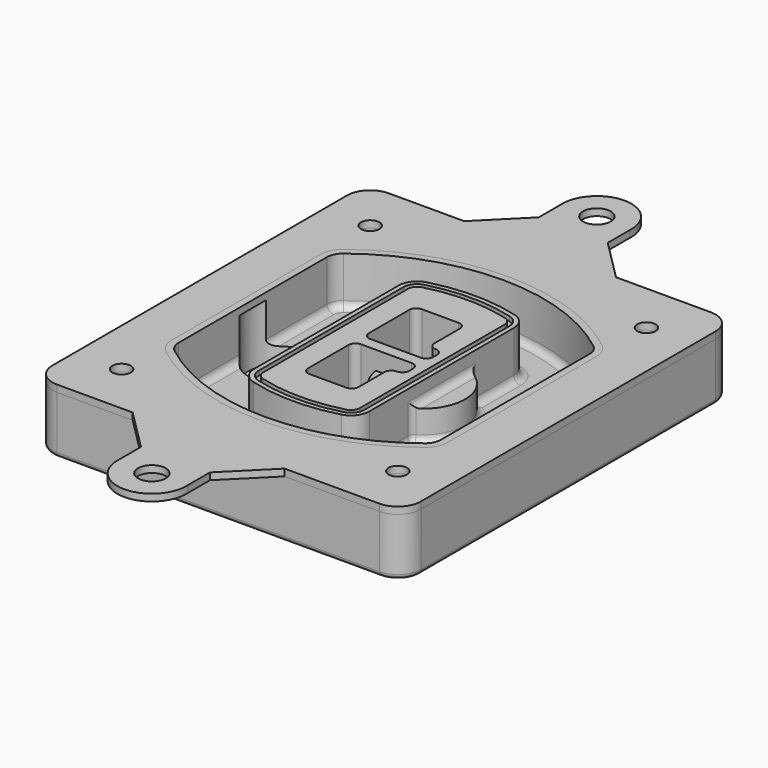
from build123d import *

# Parameters (mm, degrees)
F0_R      = 4
F1_DEPTH  = 25
F2_DEPTH  = 3
F3_DEPTH  = 18
F5_DEPTH  = 21
F6_DEPTH  = 2
F8_DEPTH  = 20
F9_DEPTH  = 16
F10_DEPTH = 25
F7_R      = 6
F7_R_2    = 4
F11_DEPTH = 6
F13_DEPTH = 9
F14_R     = 3
F15_R     = 2
F16_R     = 4
F16_R_2   = 6
F17_DEPTH = 3


# Not quite as in the source:
# - a feature names something its author has since deleted; it is built from what else it names


with BuildPart() as f1:
    # F0 (on Top) → F1 (new body)
    with BuildSketch(Plane.XY):
        with BuildLine():
            ThreePointArc((-80, -80), (-77.0710678119, -87.0710678119), (-70, -90))
            Line((-70, -90), (70, -90))
            ThreePointArc((70, -90), (77.0710678119, -87.0710678119), (80, -80))
            Line((80, -80), (80, 80))
            ThreePointArc((80, 80), (77.0710678119, 87.0710678119), (70, 90))
            Line((70, 90), (-70, 90))
            ThreePointArc((-70, 90), (-77.0710678119, 87.0710678119), (-80, 80))
            Line((-80, 80), (-80, -80))
        make_face()
        with Locations((-60, -67.5)):
            Circle(F0_R, mode=Mode.SUBTRACT)
        with Locations((60, -67.5)):
            Circle(F0_R, mode=Mode.SUBTRACT)
        with Locations((-60, 67.5)):
            Circle(F0_R, mode=Mode.SUBTRACT)
        with BuildLine():
            ThreePointArc((-64, 40.2934422872), (-62.5820384798, 46.4328484224), (-58.6153846154, 51.3286200352))
            ThreePointArc((-58.6153846154, 51.3286200352), (0, 71.5), (58.6153846154, 51.3286200352))
            ThreePointArc((58.6153846154, 51.3286200352), (62.5820384798, 46.4328484224), (64, 40.2934422872))
            Line((64, 40.2934422872), (64, -40.2934422872))
            ThreePointArc((64, -40.2934422872), (62.5820384798, -46.4328484224), (58.6153846154, -51.3286200352))
            ThreePointArc((58.6153846154, -51.3286200352), (0, -71.5), (-58.6153846154, -51.3286200352))
            ThreePointArc((-58.6153846154, -51.3286200352), (-62.5820384798, -46.4328484224), (-64, -40.2934422872))
            Line((-64, -40.2934422872), (-64, 40.2934422872))
        make_face(mode=Mode.SUBTRACT)
        with Locations((60, 67.5)):
            Circle(F0_R, mode=Mode.SUBTRACT)
        with BuildLine():
            ThreePointArc((58.6153846154, 51.3286200352), (0, 71.5), (-58.6153846154, 51.3286200352))
            ThreePointArc((-58.6153846154, 51.3286200352), (-62.5820384798, 46.4328484224), (-64, 40.2934422872))
            Line((-64, 40.2934422872), (-64, -40.2934422872))
            ThreePointArc((-64, -40.2934422872), (-62.5820384798, -46.4328484224), (-58.6153846154, -51.3286200352))
            ThreePointArc((-58.6153846154, -51.3286200352), (0, -71.5), (58.6153846154, -51.3286200352))
            ThreePointArc((58.6153846154, -51.3286200352), (62.5820384798, -46.4328484224), (64, -40.2934422872))
            Line((64, -40.2934422872), (64, 40.2934422872))
            ThreePointArc((64, 40.2934422872), (62.5820384798, 46.4328484224), (58.6153846154, 51.3286200352))
        make_face()
        with BuildLine():
            Line((-60, -40.2934422872), (-60, 40.2934422872))
            ThreePointArc((-60, 40.2934422872), (-58.9871703427, 44.6787323838), (-56.1538461538, 48.1757121072))
            ThreePointArc((-56.1538461538, 48.1757121072), (0, 67.5), (56.1538461538, 48.1757121072))
            ThreePointArc((56.1538461538, 48.1757121072), (58.9871703427, 44.6787323838), (60, 40.2934422872))
            Line((60, 40.2934422872), (60, -40.2934422872))
            ThreePointArc((60, -40.2934422872), (58.9871703427, -44.6787323838), (56.1538461538, -48.1757121072))
            ThreePointArc((56.1538461538, -48.1757121072), (0, -67.5), (-56.1538461538, -48.1757121072))
            ThreePointArc((-56.1538461538, -48.1757121072), (-58.9871703427, -44.6787323838), (-60, -40.2934422872))
        make_face(mode=Mode.SUBTRACT)
        with BuildLine():
            ThreePointArc((-56.1538461538, 48.1757121072), (-58.9871703427, 44.6787323838), (-60, 40.2934422872))
            Line((-60, 40.2934422872), (-60, -40.2934422872))
            ThreePointArc((-60, -40.2934422872), (-58.9871703427, -44.6787323838), (-56.1538461538, -48.1757121072))
            ThreePointArc((-56.1538461538, -48.1757121072), (0, -67.5), (56.1538461538, -48.1757121072))
            ThreePointArc((56.1538461538, -48.1757121072), (58.9871703427, -44.6787323838), (60, -40.2934422872))
            Line((60, -40.2934422872), (60, 40.2934422872))
            ThreePointArc((60, 40.2934422872), (58.9871703427, 44.6787323838), (56.1538461538, 48.1757121072))
            ThreePointArc((56.1538461538, 48.1757121072), (0, 67.5), (-56.1538461538, 48.1757121072))
        make_face()
        with BuildLine():
            ThreePointArc((54.3076923077, 45.8110311612), (56.2910192399, 43.3631453548), (57, 40.2934422872))
            Line((57, 40.2934422872), (57, -40.2934422872))
            ThreePointArc((57, -40.2934422872), (56.2910192399, -43.3631453548), (54.3076923077, -45.8110311612))
            ThreePointArc((54.3076923077, -45.8110311612), (0, -64.5), (-54.3076923077, -45.8110311612))
            ThreePointArc((-54.3076923077, -45.8110311612), (-56.2910192399, -43.3631453548), (-57, -40.2934422872))
            Line((-57, -40.2934422872), (-57, 40.2934422872))
            ThreePointArc((-57, 40.2934422872), (-56.2910192399, 43.3631453548), (-54.3076923077, 45.8110311612))
            ThreePointArc((-54.3076923077, 45.8110311612), (0, 64.5), (54.3076923077, 45.8110311612))
        make_face(mode=Mode.SUBTRACT)
        with BuildLine():
            Line((57, -40.2934422872), (57, 40.2934422872))
            ThreePointArc((57, 40.2934422872), (56.2910192399, 43.3631453548), (54.3076923077, 45.8110311612))
            ThreePointArc((54.3076923077, 45.8110311612), (0, 64.5), (-54.3076923077, 45.8110311612))
            ThreePointArc((-54.3076923077, 45.8110311612), (-56.2910192399, 43.3631453548), (-57, 40.2934422872))
            Line((-57, 40.2934422872), (-57, -40.2934422872))
            ThreePointArc((-57, -40.2934422872), (-56.2910192399, -43.3631453548), (-54.3076923077, -45.8110311612))
            ThreePointArc((-54.3076923077, -45.8110311612), (0, -64.5), (54.3076923077, -45.8110311612))
            ThreePointArc((54.3076923077, -45.8110311612), (56.2910192399, -43.3631453548), (57, -40.2934422872))
        make_face()
    extrude(amount=-F1_DEPTH)

    # F0 (on Top) → F2 (join)
    with BuildSketch(Plane.XY):
        with BuildLine():
            ThreePointArc((-56.1538461538, 48.1757121072), (-58.9871703427, 44.6787323838), (-60, 40.2934422872))
            Line((-60, 40.2934422872), (-60, -40.2934422872))
            ThreePointArc((-60, -40.2934422872), (-58.9871703427, -44.6787323838), (-56.1538461538, -48.1757121072))
            ThreePointArc((-56.1538461538, -48.1757121072), (0, -67.5), (56.1538461538, -48.1757121072))
            ThreePointArc((56.1538461538, -48.1757121072), (58.9871703427, -44.6787323838), (60, -40.2934422872))
            Line((60, -40.2934422872), (60, 40.2934422872))
            ThreePointArc((60, 40.2934422872), (58.9871703427, 44.6787323838), (56.1538461538, 48.1757121072))
            ThreePointArc((56.1538461538, 48.1757121072), (0, 67.5), (-56.1538461538, 48.1757121072))
        make_face()
        with BuildLine():
            ThreePointArc((54.3076923077, 45.8110311612), (56.2910192399, 43.3631453548), (57, 40.2934422872))
            Line((57, 40.2934422872), (57, -40.2934422872))
            ThreePointArc((57, -40.2934422872), (56.2910192399, -43.3631453548), (54.3076923077, -45.8110311612))
            ThreePointArc((54.3076923077, -45.8110311612), (0, -64.5), (-54.3076923077, -45.8110311612))
            ThreePointArc((-54.3076923077, -45.8110311612), (-56.2910192399, -43.3631453548), (-57, -40.2934422872))
            Line((-57, -40.2934422872), (-57, 40.2934422872))
            ThreePointArc((-57, 40.2934422872), (-56.2910192399, 43.3631453548), (-54.3076923077, 45.8110311612))
            ThreePointArc((-54.3076923077, 45.8110311612), (0, 64.5), (54.3076923077, 45.8110311612))
        make_face(mode=Mode.SUBTRACT)
    extrude(amount=F2_DEPTH)

    # F0 (on Top) → F3 (cut)
    with BuildSketch(Plane.XY):
        with BuildLine():
            Line((57, -40.2934422872), (57, 40.2934422872))
            ThreePointArc((57, 40.2934422872), (56.2910192399, 43.3631453548), (54.3076923077, 45.8110311612))
            ThreePointArc((54.3076923077, 45.8110311612), (0, 64.5), (-54.3076923077, 45.8110311612))
            ThreePointArc((-54.3076923077, 45.8110311612), (-56.2910192399, 43.3631453548), (-57, 40.2934422872))
            Line((-57, 40.2934422872), (-57, -40.2934422872))
            ThreePointArc((-57, -40.2934422872), (-56.2910192399, -43.3631453548), (-54.3076923077, -45.8110311612))
            ThreePointArc((-54.3076923077, -45.8110311612), (0, -64.5), (54.3076923077, -45.8110311612))
            ThreePointArc((54.3076923077, -45.8110311612), (56.2910192399, -43.3631453548), (57, -40.2934422872))
        make_face()
    extrude(amount=-F3_DEPTH, mode=Mode.SUBTRACT)

    # F4 (on face) → F5 (join, through all)
    with BuildSketch(Plane.XY.offset(3)):
        with BuildLine():
            ThreePointArc((-25, -39.2465276821), (-23.3511545998, -44.1109737193), (-19.0842911877, -46.9702398883))
            ThreePointArc((-19.0842911877, -46.9702398883), (0, -49.5), (19.0842911877, -46.9702398883))
            ThreePointArc((19.0842911877, -46.9702398883), (23.3511545998, -44.1109737193), (25, -39.2465276821))
            Line((25, -39.2465276821), (25, 39.2465276821))
            ThreePointArc((25, 39.2465276821), (23.3511545998, 44.1109737193), (19.0842911877, 46.9702398883))
            ThreePointArc((19.0842911877, 46.9702398883), (0, 49.5), (-19.0842911877, 46.9702398883))
            ThreePointArc((-19.0842911877, 46.9702398883), (-23.3511545998, 44.1109737193), (-25, 39.2465276821))
            Line((-25, 39.2465276821), (-25, -39.2465276821))
        make_face()
        with BuildLine():
            ThreePointArc((18.5632183908, 45.0393118368), (21.7633659499, 42.89486221), (23, 39.2465276821))
            Line((23, 39.2465276821), (23, -39.2465276821))
            ThreePointArc((23, -39.2465276821), (21.7633659499, -42.89486221), (18.5632183908, -45.0393118368))
            ThreePointArc((18.5632183908, -45.0393118368), (0, -47.5), (-18.5632183908, -45.0393118368))
            ThreePointArc((-18.5632183908, -45.0393118368), (-21.7633659499, -42.89486221), (-23, -39.2465276821))
            Line((-23, -39.2465276821), (-23, 39.2465276821))
            ThreePointArc((-23, 39.2465276821), (-21.7633659499, 42.89486221), (-18.5632183908, 45.0393118368))
            ThreePointArc((-18.5632183908, 45.0393118368), (0, 47.5), (18.5632183908, 45.0393118368))
        make_face(mode=Mode.SUBTRACT)
        with BuildLine():
            Line((23, -39.2465276821), (23, 39.2465276821))
            ThreePointArc((23, 39.2465276821), (21.7633659499, 42.89486221), (18.5632183908, 45.0393118368))
            ThreePointArc((18.5632183908, 45.0393118368), (0, 47.5), (-18.5632183908, 45.0393118368))
            ThreePointArc((-18.5632183908, 45.0393118368), (-21.7633659499, 42.89486221), (-23, 39.2465276821))
            Line((-23, 39.2465276821), (-23, -39.2465276821))
            ThreePointArc((-23, -39.2465276821), (-21.7633659499, -42.89486221), (-18.5632183908, -45.0393118368))
            ThreePointArc((-18.5632183908, -45.0393118368), (0, -47.5), (18.5632183908, -45.0393118368))
            ThreePointArc((18.5632183908, -45.0393118368), (21.7633659499, -42.89486221), (23, -39.2465276821))
        make_face()
        with BuildLine():
            ThreePointArc((18.0421455939, 43.1083837852), (20.1755772999, 41.6787507007), (21, 39.2465276821))
            Line((21, 39.2465276821), (21, -39.2465276821))
            ThreePointArc((21, -39.2465276821), (20.1755772999, -41.6787507007), (18.0421455939, -43.1083837852))
            ThreePointArc((18.0421455939, -43.1083837852), (0, -45.5), (-18.0421455939, -43.1083837852))
            ThreePointArc((-18.0421455939, -43.1083837852), (-20.1755772999, -41.6787507007), (-21, -39.2465276821))
            Line((-21, -39.2465276821), (-21, 39.2465276821))
            ThreePointArc((-21, 39.2465276821), (-20.1755772999, 41.6787507007), (-18.0421455939, 43.1083837852))
            ThreePointArc((-18.0421455939, 43.1083837852), (0, 45.5), (18.0421455939, 43.1083837852))
        make_face(mode=Mode.SUBTRACT)
        with BuildLine():
            Line((21, -39.2465276821), (21, 39.2465276821))
            ThreePointArc((21, 39.2465276821), (20.1755772999, 41.6787507007), (18.0421455939, 43.1083837852))
            ThreePointArc((18.0421455939, 43.1083837852), (0, 45.5), (-18.0421455939, 43.1083837852))
            ThreePointArc((-18.0421455939, 43.1083837852), (-20.1755772999, 41.6787507007), (-21, 39.2465276821))
            Line((-21, 39.2465276821), (-21, -39.2465276821))
            ThreePointArc((-21, -39.2465276821), (-20.1755772999, -41.6787507007), (-18.0421455939, -43.1083837852))
            ThreePointArc((-18.0421455939, -43.1083837852), (0, -45.5), (18.0421455939, -43.1083837852))
            ThreePointArc((18.0421455939, -43.1083837852), (20.1755772999, -41.6787507007), (21, -39.2465276821))
        make_face()
        with BuildLine():
            Line((-8, -2.5), (14, -2.5))
            ThreePointArc((14, -2.5), (16.1213203436, -3.3786796564), (17, -5.5))
            Line((17, -5.5), (17, -7.5))
            ThreePointArc((17, -7.5), (16.1213203436, -9.6213203436), (14, -10.5))
            ThreePointArc((14, -10.5), (11.8786796564, -11.3786796564), (11, -13.5))
            Line((11, -13.5), (11, -27.5))
            ThreePointArc((11, -27.5), (10.1213203436, -29.6213203436), (8, -30.5))
            Line((8, -30.5), (-8, -30.5))
            ThreePointArc((-8, -30.5), (-10.1213203436, -29.6213203436), (-11, -27.5))
            Line((-11, -27.5), (-11, -5.5))
            ThreePointArc((-11, -5.5), (-10.1213203436, -3.3786796564), (-8, -2.5))
        make_face(mode=Mode.SUBTRACT)
        with BuildLine():
            ThreePointArc((-8, 2.5), (-10.1213203436, 3.3786796564), (-11, 5.5))
            Line((-11, 5.5), (-11, 27.5))
            ThreePointArc((-11, 27.5), (-10.1213203436, 29.6213203436), (-8, 30.5))
            Line((-8, 30.5), (8, 30.5))
            ThreePointArc((8, 30.5), (10.1213203436, 29.6213203436), (11, 27.5))
            Line((11, 27.5), (11, 13.5))
            ThreePointArc((11, 13.5), (11.8786796564, 11.3786796564), (14, 10.5))
            ThreePointArc((14, 10.5), (16.1213203436, 9.6213203436), (17, 7.5))
            Line((17, 7.5), (17, 5.5))
            ThreePointArc((17, 5.5), (16.1213203436, 3.3786796564), (14, 2.5))
            Line((14, 2.5), (-8, 2.5))
        make_face(mode=Mode.SUBTRACT)
    extrude(amount=-F5_DEPTH)

    # F4 (on face) → F6 (cut)
    with BuildSketch(Plane.XY.offset(3)):
        with BuildLine():
            Line((23, -39.2465276821), (23, 39.2465276821))
            ThreePointArc((23, 39.2465276821), (21.7633659499, 42.89486221), (18.5632183908, 45.0393118368))
            ThreePointArc((18.5632183908, 45.0393118368), (0, 47.5), (-18.5632183908, 45.0393118368))
            ThreePointArc((-18.5632183908, 45.0393118368), (-21.7633659499, 42.89486221), (-23, 39.2465276821))
            Line((-23, 39.2465276821), (-23, -39.2465276821))
            ThreePointArc((-23, -39.2465276821), (-21.7633659499, -42.89486221), (-18.5632183908, -45.0393118368))
            ThreePointArc((-18.5632183908, -45.0393118368), (0, -47.5), (18.5632183908, -45.0393118368))
            ThreePointArc((18.5632183908, -45.0393118368), (21.7633659499, -42.89486221), (23, -39.2465276821))
        make_face()
        with BuildLine():
            ThreePointArc((18.0421455939, 43.1083837852), (20.1755772999, 41.6787507007), (21, 39.2465276821))
            Line((21, 39.2465276821), (21, -39.2465276821))
            ThreePointArc((21, -39.2465276821), (20.1755772999, -41.6787507007), (18.0421455939, -43.1083837852))
            ThreePointArc((18.0421455939, -43.1083837852), (0, -45.5), (-18.0421455939, -43.1083837852))
            ThreePointArc((-18.0421455939, -43.1083837852), (-20.1755772999, -41.6787507007), (-21, -39.2465276821))
            Line((-21, -39.2465276821), (-21, 39.2465276821))
            ThreePointArc((-21, 39.2465276821), (-20.1755772999, 41.6787507007), (-18.0421455939, 43.1083837852))
            ThreePointArc((-18.0421455939, 43.1083837852), (0, 45.5), (18.0421455939, 43.1083837852))
        make_face(mode=Mode.SUBTRACT)
    extrude(amount=-F6_DEPTH, mode=Mode.SUBTRACT)

    # F7 (on face) → F8 (join)
    with BuildSketch(Plane(origin=(0, 0, -25), x_dir=(1, 0, 0), z_dir=(0, 0, -1))):
        with BuildLine():
            ThreePointArc((3.28842436, 0), (16.7567035675, 13.4682792075), (30.224982775, 0))
            Line((30.224982775, 0), (35.224982775, 0))
            ThreePointArc((35.224982775, 0), (16.7567035675, 18.4682792075), (-1.71157564, 0))
            Line((-1.71157564, 0), (3.28842436, 0))
        make_face()
        with BuildLine():
            Line((3.28842436, 0), (30.224982775, 0))
            ThreePointArc((30.224982775, 0), (16.7567035675, 13.4682792075), (3.28842436, 0))
        make_face()
        with BuildLine():
            ThreePointArc((3.28842436, 0), (16.7567035675, -13.4682792075), (30.224982775, 0))
            Line((30.224982775, 0), (3.28842436, 0))
        make_face()
        with BuildLine():
            Line((35.224982775, 0), (30.224982775, 0))
            ThreePointArc((30.224982775, 0), (16.7567035675, -13.4682792075), (3.28842436, 0))
            Line((3.28842436, 0), (-1.71157564, 0))
            ThreePointArc((-1.71157564, 0), (16.7567035675, -18.4682792075), (35.224982775, 0))
        make_face()
    extrude(amount=-F8_DEPTH)

    # F7 (on face) → F9 (cut)
    with BuildSketch(Plane(origin=(0, 0, -25), x_dir=(1, 0, 0), z_dir=(0, 0, -1))):
        with BuildLine():
            Line((3.28842436, 0), (30.224982775, 0))
            ThreePointArc((30.224982775, 0), (16.7567035675, 13.4682792075), (3.28842436, 0))
        make_face()
        with BuildLine():
            ThreePointArc((3.28842436, 0), (16.7567035675, -13.4682792075), (30.224982775, 0))
            Line((30.224982775, 0), (3.28842436, 0))
        make_face()
    extrude(amount=-F9_DEPTH, mode=Mode.SUBTRACT)

    # F7 (on face) → F10 (cut)
    with BuildSketch(Plane(origin=(0, 0, -25), x_dir=(1, 0, 0), z_dir=(0, 0, -1))):
        with BuildLine():
            Line((-59.0318229325, 0), (-32.0952645175, 0))
            ThreePointArc((-32.0952645175, 0), (-45.563543725, 13.4682792075), (-59.0318229325, 0))
        make_face()
        with BuildLine():
            ThreePointArc((-59.0318229325, 0), (-45.563543725, -13.4682792075), (-32.0952645175, 0))
            Line((-32.0952645175, 0), (-59.0318229325, 0))
        make_face()
    extrude(amount=-F10_DEPTH, mode=Mode.SUBTRACT)

    # F7 (on face) → F11 (cut)
    with BuildSketch(Plane(origin=(0, 0, -25), x_dir=(1, 0, 0), z_dir=(0, 0, -1))):
        with Locations((60, -67.5)):
            Circle(F7_R)
        with Locations((60, -67.5)):
            Circle(F7_R_2, mode=Mode.SUBTRACT)
        with Locations((-60, -67.5)):
            Circle(F7_R)
        with Locations((-60, -67.5)):
            Circle(F7_R_2, mode=Mode.SUBTRACT)
        with Locations((-60, 67.5)):
            Circle(F7_R)
        with Locations((-60, 67.5)):
            Circle(F7_R_2, mode=Mode.SUBTRACT)
        with Locations((60, 67.5)):
            Circle(F7_R)
        with Locations((60, 67.5)):
            Circle(F7_R_2, mode=Mode.SUBTRACT)
    extrude(amount=-F11_DEPTH, mode=Mode.SUBTRACT)

    # F12 (on face) → F13 (cut, through all)
    with BuildSketch(Plane(origin=(0, 0, -9), x_dir=(1, 0, 0), z_dir=(0, 0, -1))):
        with BuildLine():
            Line((11, 13.5), (11, 17.5481537753))
            ThreePointArc((11, 17.5481537753), (2.5696536419, 11.8239143813), (-1.5415842455, 2.5))
            Line((-1.5415842455, 2.5), (3.5224848595, 2.5))
            ThreePointArc((3.5224848595, 2.5), (6.1857188154, 8.3455872281), (11.2536447004, 12.2927168648))
            ThreePointArc((11.2536447004, 12.2927168648), (11.0640958889, 12.8831798879), (11, 13.5))
        make_face()
        with BuildLine():
            ThreePointArc((11.2536447004, -12.2927168648), (6.1857188154, -8.3455872281), (3.5224848595, -2.5))
            Line((3.5224848595, -2.5), (-1.5415842455, -2.5))
            ThreePointArc((-1.5415842455, -2.5), (2.5696536419, -11.8239143813), (11, -17.5481537753))
            Line((11, -17.5481537753), (11, -13.5))
            ThreePointArc((11, -13.5), (11.0640958889, -12.8831798879), (11.2536447004, -12.2927168648))
        make_face()
        with BuildLine():
            ThreePointArc((11.2536447004, 12.2927168648), (6.1857188154, 8.3455872281), (3.5224848595, 2.5))
            Line((3.5224848595, 2.5), (14, 2.5))
            ThreePointArc((14, 2.5), (16.1213203436, 3.3786796564), (17, 5.5))
            Line((17, 5.5), (17, 7.5))
            ThreePointArc((17, 7.5), (16.1213203436, 9.6213203436), (14, 10.5))
            ThreePointArc((14, 10.5), (12.3601599782, 10.9878446101), (11.2536447004, 12.2927168648))
        make_face()
        with BuildLine():
            Line((14, -2.5), (3.5224848595, -2.5))
            ThreePointArc((3.5224848595, -2.5), (6.1857188154, -8.3455872281), (11.2536447004, -12.2927168648))
            ThreePointArc((11.2536447004, -12.2927168648), (12.3601599782, -10.9878446101), (14, -10.5))
            ThreePointArc((14, -10.5), (16.1213203436, -9.6213203436), (17, -7.5))
            Line((17, -7.5), (17, -5.5))
            ThreePointArc((17, -5.5), (16.1213203436, -3.3786796564), (14, -2.5))
        make_face()
    extrude(amount=F13_DEPTH, mode=Mode.SUBTRACT)

    # F14
    f14_edges = [f1.edges().sort_by_distance(p)[0] for p in [
        (-57, -23.703476, -18),
        (-57, 23.703476, -18),
        (25, 0, -5),
        (25, 16.526506, -11.5),
        (25, -16.526506, -11.5),
        (25, -27.886517, -18),
        (35.224983, 0, -18),
    ]]
    fillet(f14_edges, radius=F14_R)

    # F15
    f15_edges = [f1.edges().sort_by_distance(p)[0] for p in [
        (0, -90, -25),
    ]]
    fillet(f15_edges, radius=F15_R)


with BuildPart() as f17:
    # F16 (on face) → F17 (new body, through all)
    with BuildSketch(Plane.XY):
        with BuildLine():
            Line((70, 90), (28.7904447417, 90))
            Line((28.7904447417, 90), (-37.1657916524, 90))
            Line((-37.1657916524, 90), (-70, 90))
            ThreePointArc((-70, 90), (-77.0710678119, 87.0710678119), (-80, 80))
            Line((-80, 80), (-80, -80))
            ThreePointArc((-80, -80), (-77.0710678119, -87.0710678119), (-70, -90))
            Line((-70, -90), (-37.1657916524, -90))
            Line((-37.1657916524, -90), (28.7904447417, -90))
            Line((28.7904447417, -90), (70, -90))
            ThreePointArc((70, -90), (77.0710678119, -87.0710678119), (80, -80))
            Line((80, -80), (80, 80))
            ThreePointArc((80, 80), (77.0710678119, 87.0710678119), (70, 90))
        make_face()
        with Locations((-60, -67.5)):
            Circle(F16_R, mode=Mode.SUBTRACT)
        with Locations((60, -67.5)):
            Circle(F16_R, mode=Mode.SUBTRACT)
        with Locations((-60, 67.5)):
            Circle(F16_R, mode=Mode.SUBTRACT)
        with BuildLine():
            ThreePointArc((-60, 40.2934422872), (-58.9871703427, 44.6787323838), (-56.1538461538, 48.1757121072))
            ThreePointArc((-56.1538461538, 48.1757121072), (0, 67.5), (56.1538461538, 48.1757121072))
            ThreePointArc((56.1538461538, 48.1757121072), (58.9871703427, 44.6787323838), (60, 40.2934422872))
            Line((60, 40.2934422872), (60, -40.2934422872))
            ThreePointArc((60, -40.2934422872), (58.9871703427, -44.6787323838), (56.1538461538, -48.1757121072))
            ThreePointArc((56.1538461538, -48.1757121072), (0, -67.5), (-56.1538461538, -48.1757121072))
            ThreePointArc((-56.1538461538, -48.1757121072), (-58.9871703427, -44.6787323838), (-60, -40.2934422872))
            Line((-60, -40.2934422872), (-60, 40.2934422872))
        make_face(mode=Mode.SUBTRACT)
        with Locations((60, 67.5)):
            Circle(F16_R, mode=Mode.SUBTRACT)
        with BuildLine():
            Line((10.7904447417, 108), (10.7904447417, 120))
            ThreePointArc((10.7904447417, 120), (-4.1876734553, 135.8099230061), (-19.1657916524, 120))
            Line((-19.1657916524, 120), (-19.1657916524, 108))
            Line((-19.1657916524, 108), (-37.1657916524, 90))
            Line((-37.1657916524, 90), (28.7904447417, 90))
            Line((28.7904447417, 90), (10.7904447417, 108))
        make_face()
        with Locations((-4.1876734553, 120.8099230061)):
            Circle(F16_R_2, mode=Mode.SUBTRACT)
        with BuildLine():
            Line((10.7904447417, -108), (28.7904447417, -90))
            Line((28.7904447417, -90), (-37.1657916524, -90))
            Line((-37.1657916524, -90), (-19.1657916524, -108))
            Line((-19.1657916524, -108), (-19.1657916524, -120))
            ThreePointArc((-19.1657916524, -120), (-4.1876734553, -135.8099230061), (10.7904447417, -120))
            Line((10.7904447417, -120), (10.7904447417, -108))
        make_face()
        with Locations((-4.1876734553, -120.8099230061)):
            Circle(F16_R_2, mode=Mode.SUBTRACT)
    extrude(amount=F17_DEPTH)


solid = Compound([f1.part, f17.part])
